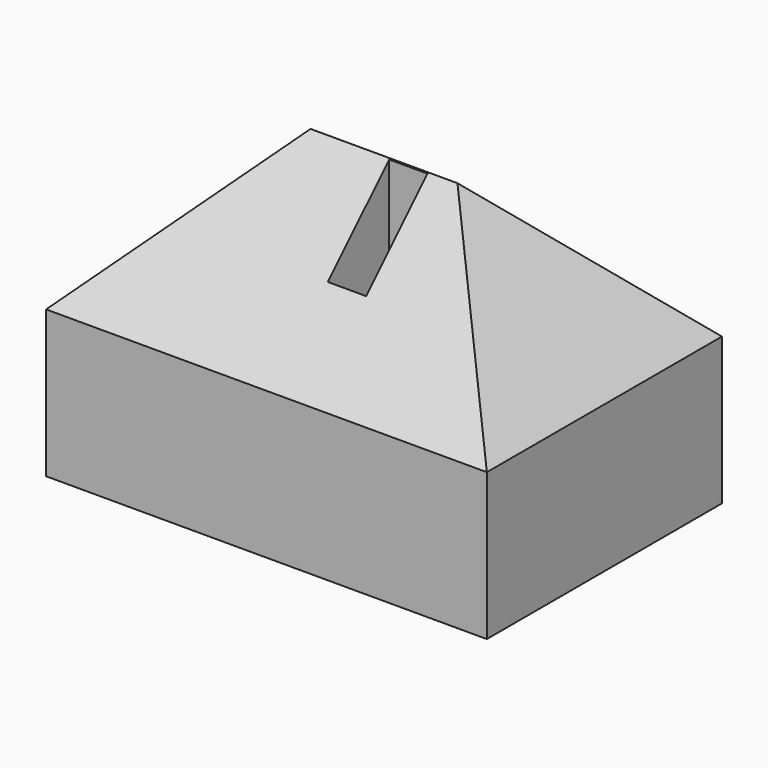
from build123d import *

# Parameters (mm, degrees)
F0_W     = 76.2
F0_H     = 50.8
F1_DEPTH = 50.8
F3_SIZE  = 25.39999
F4_W     = 6.6249594092
F4_H     = 13.2540166378
F5_DEPTH = 50.801


# Not quite as in the source:
# - a fillet or chamfer is up to 0.001 mm smaller than in the source, because OpenCascade refuses the exact size


with BuildPart() as f1:
    # F0 (on Top) → F1 (new body)
    with BuildSketch(Plane.XY):
        with Locations((38.1, 25.4)):
            Rectangle(F0_W, F0_H)
    extrude(amount=F1_DEPTH)

    # F3 (size 25.4 in the source; OpenCascade refuses exactly that, so slightly less here)
    f3_edges = [f1.edges().sort_by_distance(p)[0] for p in [
        (0, 25.4, 50.8),
        (76.2, 25.4, 50.8),
        (38.1, 0, 50.8),
        (38.1, 50.8, 50.8),
    ]]
    chamfer(f3_edges, length=F3_SIZE)

    # F4 (on face) → F5 (cut, through all)
    with BuildSketch(Plane(origin=(0, 0, 0), x_dir=(1, 0, 0), z_dir=(0, 0, -1))):
        with Locations((42.4170047045, -18.6321474612)):
            Rectangle(F4_W, F4_H)
    extrude(amount=-F5_DEPTH, mode=Mode.SUBTRACT)


solid = f1.part
